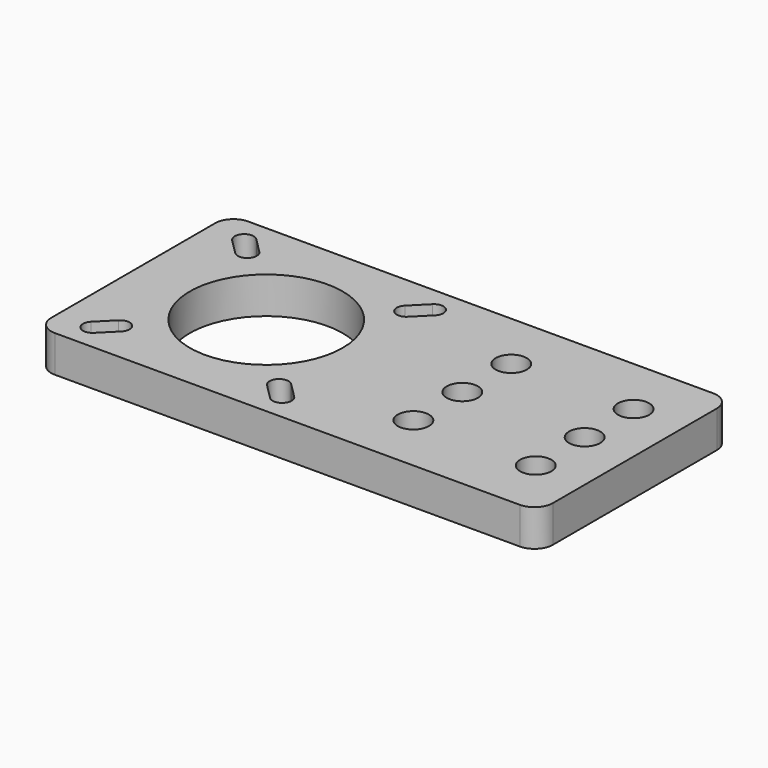
from build123d import *

# Parameters (mm, degrees)
F0_R     = 12.5
F0_R_2   = 2.55
F1_DEPTH = 6


# Not quite as in the source:
# - ends of sketch curves that miss each other by under 0.0002 mm in the source are joined


with BuildPart() as f1:
    # F0 (on Top) → F1 (new body)
    with BuildSketch(Plane.XY):
        with BuildLine():
            Line((38, 19.75), (-38, 19.75))
            ThreePointArc((-38, 19.75), (-40.1213203436, 18.8713203436), (-41, 16.75))
            Line((-41, 16.75), (-41, -16.75))
            ThreePointArc((-41, -16.75), (-40.1213203436, -18.8713203436), (-38, -19.75))
            Line((-38, -19.75), (38, -19.75))
            ThreePointArc((38, -19.75), (40.1213203436, -18.8713203436), (41, -16.75))
            Line((41, -16.75), (41, 16.75))
            ThreePointArc((41, 16.75), (40.1213203436, 18.8713203436), (38, 19.75))
        make_face()
        with BuildLine():
            ThreePointArc((-34.1539839892, -16.5960150108), (-36.3460155108, -16.5960155108), (-36.3460150108, -14.4039839892))
            Line((-36.346015, -14.403984), (-33.846015, -11.903984))
            ThreePointArc((-33.8460150108, -11.9039839892), (-31.6539844892, -11.9039844892), (-31.6539839892, -14.0960150108))
            Line((-31.653984, -14.096015), (-34.153984, -16.596015))
        make_face(mode=Mode.SUBTRACT)
        with BuildLine():
            ThreePointArc((-3.1539844892, -14.4039844892), (-3.1539844892, -16.5960155108), (-5.3460155108, -16.5960155108))
            Line((-5.3460155108, -16.5960155108), (-7.846015, -14.096015))
            ThreePointArc((-7.846015, -14.096015), (-7.8460155108, -11.9039844892), (-5.6539844892, -11.9039844892))
            Line((-5.6539844892, -11.9039844892), (-3.1539844892, -14.4039844892))
        make_face(mode=Mode.SUBTRACT)
        with Locations((-19.25, 0)):
            Circle(F0_R, mode=Mode.SUBTRACT)
        with Locations((12.8, -10)):
            Circle(F0_R_2, mode=Mode.SUBTRACT)
        with Locations((32.8, -10)):
            Circle(F0_R_2, mode=Mode.SUBTRACT)
        with Locations((12.8, 0)):
            Circle(F0_R_2, mode=Mode.SUBTRACT)
        with Locations((32.8, 0)):
            Circle(F0_R_2, mode=Mode.SUBTRACT)
        with BuildLine():
            ThreePointArc((-31.6539844892, 14.0960155108), (-31.6539844892, 11.9039844892), (-33.8460155108, 11.9039844892))
            Line((-33.8460155108, 11.9039844892), (-36.346015, 14.403985))
            ThreePointArc((-36.346015, 14.403985), (-36.3460155108, 16.5960155108), (-34.1539844892, 16.5960155108))
            Line((-34.1539844892, 16.5960155108), (-31.6539844892, 14.0960155108))
        make_face(mode=Mode.SUBTRACT)
        with BuildLine():
            ThreePointArc((-5.3460150108, 16.5960160108), (-3.1539844892, 16.5960155108), (-3.1539839892, 14.4039849892))
            Line((-3.153984, 14.403985), (-5.653984, 11.903985))
            ThreePointArc((-5.6539839892, 11.9039849892), (-7.8460155108, 11.9039844892), (-7.8460150108, 14.0960160108))
            Line((-7.846015, 14.096016), (-5.346015, 16.596016))
        make_face(mode=Mode.SUBTRACT)
        with Locations((12.8, 10)):
            Circle(F0_R_2, mode=Mode.SUBTRACT)
        with Locations((32.8, 10)):
            Circle(F0_R_2, mode=Mode.SUBTRACT)
    extrude(amount=F1_DEPTH)


solid = f1.part
